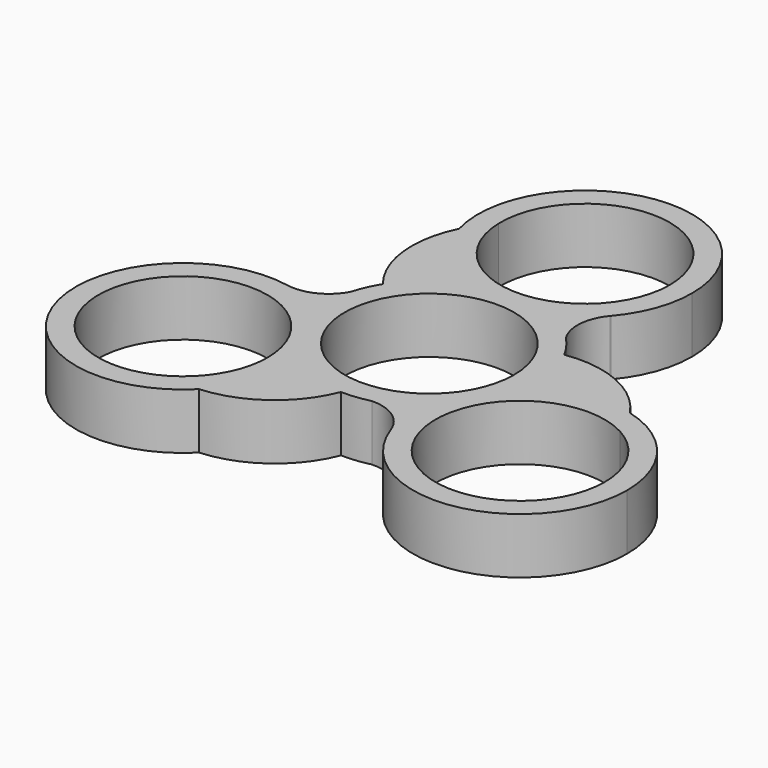
from build123d import *

# Parameters (mm, degrees)
F0_R     = 11.049
F1_DEPTH = 7.2898


# Not quite as in the source:
# - a feature names something its author has since deleted; it is built from what else it names


with BuildPart() as f1:
    # F0 (on Top) → F1 (new body)
    with BuildSketch(Plane.XY):
        with BuildLine():
            ThreePointArc((13.9084581944, -1.3098437524), (13.9546060671, -0.655644349), (13.97, 0))
            ThreePointArc((13.97, 0), (13.5399902372, 3.4394133768), (12.2764331601, 6.6670899848))
            ThreePointArc((12.2764331601, 6.6670899848), (11.2762217496, 8.2466795168), (10.0740419848, 9.6785628111))
            ThreePointArc((10.0740419848, 9.6785628111), (8.0892761862, 11.3896668425), (5.8198711326, 12.7))
            ThreePointArc((5.8198711326, 12.7), (0, 11.43), (-5.8198711326, 12.7))
            ThreePointArc((-5.8198711326, 12.7), (-9.2682549118, 10.4527676187), (-11.9120858762, 7.2981579921))
            ThreePointArc((-11.9120858762, 7.2981579921), (-12.7799448333, 5.6421547355), (-13.4189022589, 3.8850948721))
            ThreePointArc((-13.4189022589, 3.8850948721), (-13.9083789193, 1.3106852543), (-13.9084581944, -1.3098437524))
            ThreePointArc((-13.9084581944, -1.3098437524), (-9.8986703653, -5.715), (-8.0885870618, -11.3901562476))
            ThreePointArc((-8.0885870618, -11.3901562476), (-4.4182348417, -13.2529280117), (-0.3643472839, -13.9652479769))
            ThreePointArc((-0.3643472839, -13.9652479769), (1.5037230836, -13.8888342523), (3.3448602741, -13.5636576832))
            ThreePointArc((3.3448602741, -13.5636576832), (5.8191027331, -12.7003520968), (8.0885870618, -11.3901562476))
            ThreePointArc((8.0885870618, -11.3901562476), (9.8986703653, -5.715), (13.9084581944, -1.3098437524))
        make_face()
        Circle(F0_R, mode=Mode.SUBTRACT)
        with BuildLine():
            ThreePointArc((12.2764331601, 6.6670899848), (13.5399902372, 3.4394133768), (13.97, 0))
            ThreePointArc((13.97, 0), (13.9546060671, -0.655644349), (13.9084581944, -1.3098437524))
            ThreePointArc((13.9084581944, -1.3098437524), (19.4758239296, 1.0406092668), (25.5149823418, 0.8198009845))
            ThreePointArc((25.5149823418, 0.8198009845), (19.7483617265, 5.673895919), (12.2764331601, 6.6670899848))
        make_face()
        with BuildLine():
            ThreePointArc((25.5149823418, 0.8198009845), (19.4758239296, 1.0406092668), (13.9084581944, -1.3098437524))
            ThreePointArc((13.9084581944, -1.3098437524), (12.0983748909, -6.985), (8.0885870618, -11.3901562476))
            ThreePointArc((8.0885870618, -11.3901562476), (8.1283324688, -14.3791979101), (8.8030929872, -17.2913531259))
            ThreePointArc((8.8030929872, -17.2913531259), (8.8153498636, -17.3259186272), (8.8273812481, -17.3605632616))
            ThreePointArc((8.8273812481, -17.3605632616), (24.3614367008, -26.4684622633), (35.9670452561, -12.7))
            ThreePointArc((35.9670452561, -12.7), (33.0493409698, -4.1555480306), (25.5149823418, 0.8198009845))
        make_face()
        with BuildLine():
            ThreePointArc((33.0460452561, -12.7), (12.502346623, -18.3507609104), (27.2661377773, -2.9883026713))
            ThreePointArc((27.2661377773, -2.9883026713), (31.4917438892, -7.0492390896), (33.0460452561, -12.7))
        make_face(mode=Mode.SUBTRACT)
        with BuildLine():
            ThreePointArc((8.0885870618, -11.3901562476), (12.0983748909, -6.985), (13.9084581944, -1.3098437524))
            ThreePointArc((13.9084581944, -1.3098437524), (9.8986703653, -5.715), (8.0885870618, -11.3901562476))
        make_face()
        with BuildLine():
            ThreePointArc((5.8198711326, 12.7), (8.0892761862, 11.3896668425), (10.0740419848, 9.6785628111))
            ThreePointArc((10.0740419848, 9.6785628111), (9.2542217215, 13.054963054), (10.5732045792, 16.2693787218))
            ThreePointArc((10.5732045792, 16.2693787218), (8.3885844419, 14.2289413634), (5.8198711326, 12.7))
        make_face()
        with BuildLine():
            ThreePointArc((8.8030929872, -17.2913531259), (8.1283324688, -14.3791979101), (8.0885870618, -11.3901562476))
            ThreePointArc((8.0885870618, -11.3901562476), (5.8191027331, -12.7003520968), (3.3448602741, -13.5636576832))
            ThreePointArc((3.3448602741, -13.5636576832), (6.6788187895, -14.54187263), (8.8030929872, -17.2913531259))
        make_face()
        with BuildLine():
            ThreePointArc((-5.8198711326, 12.7), (0, 11.43), (5.8198711326, 12.7))
            ThreePointArc((5.8198711326, 12.7), (0, 13.97), (-5.8198711326, 12.7))
        make_face()
        with BuildLine():
            ThreePointArc((-5.8198711326, 12.7), (0, 13.97), (5.8198711326, 12.7))
            ThreePointArc((5.8198711326, 12.7), (8.3885844419, 14.2289413634), (10.5732045792, 16.2693787218))
            ThreePointArc((10.5732045792, 16.2693787218), (10.5970107433, 16.2972762387), (10.6209981845, 16.3250180405))
            ThreePointArc((10.6209981845, 16.3250180405), (13.1060338134, 20.563391924), (13.97, 25.4))
            ThreePointArc((13.97, 25.4), (-1.87356461, 39.2437948429), (-13.4674596495, 21.6867223928))
            ThreePointArc((-13.4674596495, 21.6867223928), (-10.6391060252, 16.3462536492), (-5.8198711326, 12.7))
        make_face()
        with BuildLine():
            ThreePointArc((11.049, 25.4), (0.1463531826, 14.3519693273), (-11.0451228611, 25.1073193139))
            ThreePointArc((-11.0451228611, 25.1073193139), (-0.1463531826, 36.4480306727), (11.049, 25.4))
        make_face(mode=Mode.SUBTRACT)
        with BuildLine():
            ThreePointArc((8.8273812481, -17.3605632616), (8.8153498636, -17.3259186272), (8.8030929872, -17.2913531259))
            ThreePointArc((8.8030929872, -17.2913531259), (8.8151916949, -17.3259741342), (8.8273812481, -17.3605632616))
        make_face()
        with BuildLine():
            ThreePointArc((-11.9120858762, 7.2981579921), (-9.2682549118, 10.4527676187), (-5.8198711326, 12.7))
            ThreePointArc((-5.8198711326, 12.7), (-10.6391060252, 16.3462536492), (-13.4674596495, 21.6867223928))
            ThreePointArc((-13.4674596495, 21.6867223928), (-14.7879188675, 14.2656349788), (-11.9120858762, 7.2981579921))
        make_face()
        with BuildLine():
            ThreePointArc((-12.0475226922, -22.5065233774), (-4.960442859, -19.9395308977), (-0.3643472839, -13.9652479769))
            ThreePointArc((-0.3643472839, -13.9652479769), (-4.4182348417, -13.2529280117), (-8.0885870618, -11.3901562476))
            ThreePointArc((-8.0885870618, -11.3901562476), (-8.042439189, -12.044355651), (-8.0270452561, -12.7))
            ThreePointArc((-8.0270452561, -12.7), (-9.0711849324, -17.9993428735), (-12.0475226922, -22.5065233774))
        make_face()
        with BuildLine():
            ThreePointArc((-8.0270452561, -12.7), (-8.042439189, -12.044355651), (-8.0885870618, -11.3901562476))
            ThreePointArc((-8.0885870618, -11.3901562476), (-12.0983748909, -6.985), (-13.9084581944, -1.3098437524))
            ThreePointArc((-13.9084581944, -1.3098437524), (-16.5169169106, 0.1502565467), (-19.3762975665, 1.0219744041))
            ThreePointArc((-19.3762975665, 1.0219744041), (-19.4123606069, 1.0286423885), (-19.4483794326, 1.0355452211))
            ThreePointArc((-19.4483794326, 1.0355452211), (-35.3240264115, -16.8895671954), (-12.0475226922, -22.5065233774))
            ThreePointArc((-12.0475226922, -22.5065233774), (-9.0711849324, -17.9993428735), (-8.0270452561, -12.7))
        make_face()
        with BuildLine():
            ThreePointArc((-10.9480452561, -12.7), (-12.3559934404, -18.0972697623), (-16.2210149162, -22.1190166425))
            ThreePointArc((-16.2210149162, -22.1190166425), (-31.6380970718, -7.3027302377), (-10.9480452561, -12.7))
        make_face(mode=Mode.SUBTRACT)
        with BuildLine():
            ThreePointArc((-13.9084581944, -1.3098437524), (-12.0983748909, -6.985), (-8.0885870618, -11.3901562476))
            ThreePointArc((-8.0885870618, -11.3901562476), (-9.8986703653, -5.715), (-13.9084581944, -1.3098437524))
        make_face()
        with BuildLine():
            ThreePointArc((-13.9084581944, -1.3098437524), (-13.9083789193, 1.3106852543), (-13.4189022589, 3.8850948721))
            ThreePointArc((-13.4189022589, 3.8850948721), (-15.933040511, 1.486909576), (-19.3762975665, 1.0219744041))
            ThreePointArc((-19.3762975665, 1.0219744041), (-16.5169169106, 0.1502565467), (-13.9084581944, -1.3098437524))
        make_face()
        with BuildLine():
            ThreePointArc((-19.3762975665, 1.0219744041), (-19.412329593, 1.0288071201), (-19.4483794326, 1.0355452211))
            ThreePointArc((-19.4483794326, 1.0355452211), (-19.4123606069, 1.0286423885), (-19.3762975665, 1.0219744041))
        make_face()
    extrude(amount=F1_DEPTH)


solid = f1.part
